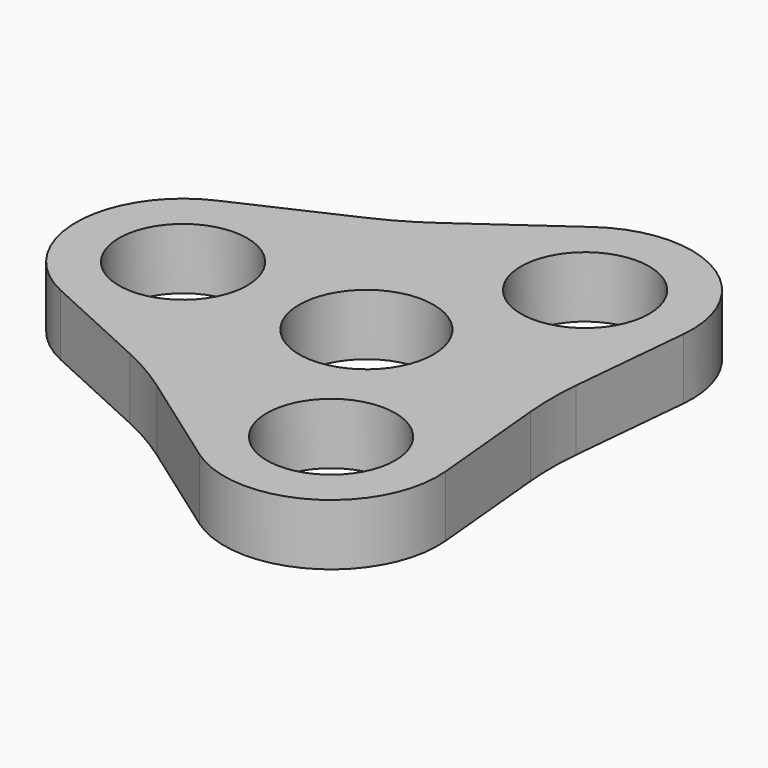
from build123d import *

# Parameters (mm, degrees)
F0_R     = 11
F1_DEPTH = 10
F2_COUNT = 3
F4_R     = 10.5
F5_DEPTH = 25
F6_R     = 50
F7_T     = -2


with BuildPart() as f1:
    # F0 (on Top) → F1 (new body)
    with BuildSketch(Plane.XY):
        with BuildLine():
            Line((-12.5, 27.2717802866), (-37.2916666667, 15.9085385005))
            ThreePointArc((-37.2916666667, 15.9085385005), (-47.5, 0), (-37.2916666667, -15.9085385005))
            Line((-37.2916666667, -15.9085385005), (-12.5, -27.2717802866))
            ThreePointArc((-12.5, -27.2717802866), (30, 0), (-12.5, 27.2717802866))
        make_face()
        Circle(F0_R, mode=Mode.SUBTRACT)
    extrude(amount=F1_DEPTH)


with BuildPart() as f2_1:
    # F2: instance of F1
    add(f1.part.rotate(Axis((0, 0, 0), (0, 0, -1)), 1 * 360 / F2_COUNT))


with BuildPart() as f2_2:
    # F2: instance of F1
    add(f1.part.rotate(Axis((0, 0, 0), (0, 0, -1)), 2 * 360 / F2_COUNT))


with BuildPart() as f1_1:
    add(f1.part)

    # F3: union F2_1, F2_2
    add(f2_1.part)
    add(f2_2.part)

    # F4 (on face) → F5 (cut)
    with BuildSketch(Plane.XY.offset(10)):
        with Locations((15, 25.9807621135)):
            Circle(F4_R)
        with Locations((15, -25.9807621135)):
            Circle(F4_R)
        with Locations((-30, 0)):
            Circle(F4_R)
    extrude(amount=-F5_DEPTH, mode=Mode.SUBTRACT)

    # F6
    f6_edges = [f1_1.edges().sort_by_distance(p)[0] for p in [
        (-15.066264, -26.095535, 5),
        (-15.066264, 26.095535, 5),
        (30.132528, 0, 5),
    ]]
    fillet(f6_edges, radius=F6_R)

    # F7
    f7_openings = [f1_1.faces().sort_by_distance(p)[0] for p in [
        (-27.825176, 18.947668, 0),
    ]]
    offset(amount=F7_T, openings=f7_openings)


solid = f1_1.part
